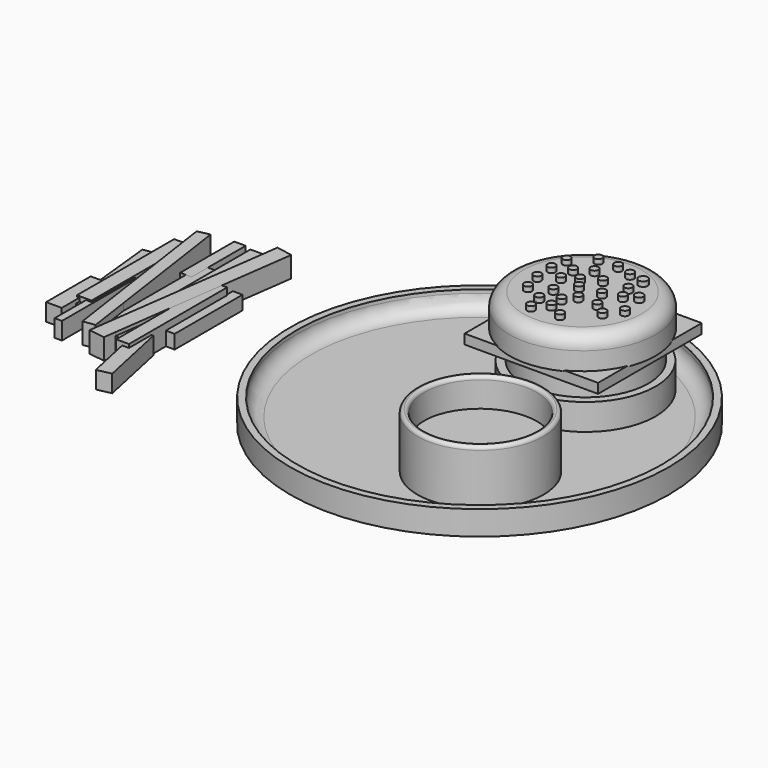
from build123d import *

# Parameters (mm, degrees)
F0_R      = 69.415848621
F1_DEPTH  = 8.89
F2_T      = -2.54
F3_R      = 5.08
F4_R      = 25.7769025516
F5_DEPTH  = 12.192
F6_R      = 22.9963503977
F7_DEPTH  = 19.05
F9_START  = 19.304
F8_W      = 48.926981166
F8_H      = 47.4879527465
F9_DEPTH  = 3.556
F11_START = 22.606
F10_R     = 26.7992090527
F11_DEPTH = 11.938
F12_R     = 5.08
F13_R     = 1.4675266157
F14_DEPTH = 36.322
F13_R_2   = 1.4390293509
F13_R_3   = 1.6781766258
F13_R_4   = 1.5498825968
F15_R     = 23.1464516615
F16_DEPTH = 22.606
F17_T     = 2.54
F18_R     = 21.0117914826
F19_DEPTH = 12.192
F20_R     = 1.26999
F22_DEPTH = 6.35
F21_W     = 0.3085602075
F21_H     = 28.0814692059
F23_DEPTH = 7.62
F24_DEPTH = 5.08
F25_DEPTH = 7.62
F26_DEPTH = 6.35
F21_W_2   = 2.106167376
F21_H_2   = 7.4712689966
F27_DEPTH = 5.08
F28_DEPTH = 5.08
F29_DEPTH = 7.62
F21_W_3   = 0.9008161724
F21_H_3   = 12.3305870922
F30_DEPTH = 6.858
F31_DEPTH = 6.35
F32_DEPTH = 5.08
F33_DEPTH = 6.35


# Not quite as in the source:
# - a fillet or chamfer is up to 0.001 mm smaller than in the source, because OpenCascade refuses the exact size
# - a shell that OpenCascade refuses in one call is made with other operations: the cavity is built on its own and cut out


with BuildPart() as f1:
    # F0 (on Top) → F1 (new body)
    with BuildSketch(Plane.XY):
        Circle(F0_R)
    extrude(amount=F1_DEPTH)

    # F2
    f2_openings = [f1.faces().sort_by_distance(p)[0] for p in [
        (0, 0, 8.89),
    ]]
    offset(amount=F2_T, openings=f2_openings)

    # F3
    f3_edges = [f1.edges().sort_by_distance(p)[0] for p in [
        (-66.875849, 0, 2.54),
    ]]
    fillet(f3_edges, radius=F3_R)

    # F4 (on Top) → F5 (join)
    with BuildSketch(Plane.XY):
        with Locations((13.4006887674, 31.7715257406)):
            Circle(F4_R)
    extrude(amount=F5_DEPTH)

    # F6 (on Top) → F7 (join)
    with BuildSketch(Plane.XY):
        with Locations((13.4006887674, 31.9251716137)):
            Circle(F6_R)
    extrude(amount=F7_DEPTH)

    # F15 (on Top) → F16 (join)
    with BuildSketch(Plane.XY):
        with Locations((21.2976261973, -26.1903237551)):
            Circle(F15_R)
    extrude(amount=F16_DEPTH)

    # F17: shell of thickness 2.54, made by hand


with BuildPart() as f9:
    # F8 (on Top) → F9 (new body)
    with BuildSketch(Plane.XY.offset(F9_START)):
        with Locations((13.2390661165, 30.9391203336)):
            Rectangle(F8_W, F8_H)
    extrude(amount=F9_DEPTH)


with BuildPart() as f11:
    # F10 (on Top) → F11 (new body)
    with BuildSketch(Plane.XY.offset(F11_START)):
        with Locations((13.0065530539, 30.9398267418)):
            Circle(F10_R)
    extrude(amount=F11_DEPTH)

    # F12
    f12_edges = [f11.edges().sort_by_distance(p)[0] for p in [
        (-13.792656, 30.939827, 34.544),
    ]]
    fillet(f12_edges, radius=F12_R)


with BuildPart() as f14:
    # F13 (on Top) → F14 (new body)
    with BuildSketch(Plane.XY):
        with Locations((0, 22.1610423177)):
            Circle(F13_R)
    extrude(amount=F14_DEPTH)


with BuildPart() as f14b:
    # F13 (on Top) → F14, piece 2 (new body)
    with BuildSketch(Plane.XY):
        with Locations((12.3756462708, 22.1610423177)):
            Circle(F13_R_2)
    extrude(amount=F14_DEPTH)


with BuildPart() as f14c:
    # F13 (on Top) → F14, piece 3 (new body)
    with BuildSketch(Plane.XY):
        with Locations((6.7634354346, 25.4012537548)):
            Circle(F13_R_2)
    extrude(amount=F14_DEPTH)


with BuildPart() as f14d:
    # F13 (on Top) → F14, piece 4 (new body)
    with BuildSketch(Plane.XY):
        with Locations((6.7634354346, 18.9208308807)):
            Circle(F13_R_2)
    extrude(amount=F14_DEPTH)


with BuildPart() as f14e:
    # F13 (on Top) → F14, piece 5 (new body)
    with BuildSketch(Plane.XY):
        with Locations((11.4056941927, 31.3545369015)):
            Circle(F13_R_2)
    extrude(amount=F14_DEPTH)


with BuildPart() as f14f:
    # F13 (on Top) → F14, piece 6 (new body)
    with BuildSketch(Plane.XY):
        with Locations((3.9288703727, 32.3982093437)):
            Circle(F13_R_2)
    extrude(amount=F14_DEPTH)


with BuildPart() as f14g:
    # F13 (on Top) → F14, piece 7 (new body)
    with BuildSketch(Plane.XY):
        with Locations((19.0983680662, 32.2760957669)):
            Circle(F13_R_2)
    extrude(amount=F14_DEPTH)


with BuildPart() as f14h:
    # F13 (on Top) → F14, piece 8 (new body)
    with BuildSketch(Plane.XY):
        with Locations((14.453937741, 38.4773673317)):
            Circle(F13_R_2)
    extrude(amount=F14_DEPTH)


with BuildPart() as f14i:
    # F13 (on Top) → F14, piece 9 (new body)
    with BuildSketch(Plane.XY):
        with Locations((15.2537068352, 26.1903237551)):
            Circle(F13_R_2)
    extrude(amount=F14_DEPTH)


with BuildPart() as f14j:
    # F13 (on Top) → F14, piece 10 (new body)
    with BuildSketch(Plane.XY):
        with Locations((22.4464706145, 25.903635466)):
            Circle(F13_R_2)
    extrude(amount=F14_DEPTH)


with BuildPart() as f14k:
    # F13 (on Top) → F14, piece 11 (new body)
    with BuildSketch(Plane.XY):
        with Locations((-2.0858600398, 35.5903968791)):
            Circle(F13_R_2)
    extrude(amount=F14_DEPTH)


with BuildPart() as f14l:
    # F13 (on Top) → F14, piece 12 (new body)
    with BuildSketch(Plane.XY):
        with Locations((-1.8430103329, 28.7853937772)):
            Circle(F13_R_2)
    extrude(amount=F14_DEPTH)


with BuildPart() as f14m:
    # F13 (on Top) → F14, piece 13 (new body)
    with BuildSketch(Plane.XY):
        with Locations((8.7462493805, 41.772702743)):
            Circle(F13_R_2)
    extrude(amount=F14_DEPTH)


with BuildPart() as f14n:
    # F13 (on Top) → F14, piece 14 (new body)
    with BuildSketch(Plane.XY):
        with Locations((8.7462493805, 35.1820319203)):
            Circle(F13_R_2)
    extrude(amount=F14_DEPTH)


with BuildPart() as f14o:
    # F13 (on Top) → F14, piece 15 (new body)
    with BuildSketch(Plane.XY):
        with Locations((3.6562509812, 38.3103937772)):
            Circle(F13_R_2)
    extrude(amount=F14_DEPTH)


with BuildPart() as f14p:
    # F13 (on Top) → F14, piece 16 (new body)
    with BuildSketch(Plane.XY):
        with Locations((-1.5703909413, 41.9232093437)):
            Circle(F13_R_2)
    extrude(amount=F14_DEPTH)


with BuildPart() as f14q:
    # F13 (on Top) → F14, piece 17 (new body)
    with BuildSketch(Plane.XY):
        with Locations((18.0482084397, 14.3602699913)):
            Circle(F13_R_2)
    extrude(amount=F14_DEPTH)


with BuildPart() as f14r:
    # F13 (on Top) → F14, piece 18 (new body)
    with BuildSketch(Plane.XY):
        with Locations((26.8960847251, 22.6954062536)):
            Circle(F13_R_2)
    extrude(amount=F14_DEPTH)


with BuildPart() as f14s:
    # F13 (on Top) → F14, piece 19 (new body)
    with BuildSketch(Plane.XY):
        with Locations((8.2464414958, 13.2429551706)):
            Circle(F13_R_2)
    extrude(amount=F14_DEPTH)


with BuildPart() as f14t:
    # F13 (on Top) → F14, piece 20 (new body)
    with BuildSketch(Plane.XY):
        with Locations((12.4221230696, 17.3662139487)):
            Circle(F13_R_2)
    extrude(amount=F14_DEPTH)


with BuildPart() as f14u:
    # F13 (on Top) → F14, piece 21 (new body)
    with BuildSketch(Plane.XY):
        with Locations((12.3846795339, 48.0746486285)):
            Circle(F13_R_2)
    extrude(amount=F14_DEPTH)


with BuildPart() as f14v:
    # F13 (on Top) → F14, piece 22 (new body)
    with BuildSketch(Plane.XY):
        with Locations((5.1078192271, 48.0746486285)):
            Circle(F13_R_2)
    extrude(amount=F14_DEPTH)


with BuildPart() as f14w:
    # F13 (on Top) → F14, piece 23 (new body)
    with BuildSketch(Plane.XY):
        with Locations((23.118837317, 39.3239505656)):
            Circle(F13_R_2)
    extrude(amount=F14_DEPTH)


with BuildPart() as f14x:
    # F13 (on Top) → F14, piece 24 (new body)
    with BuildSketch(Plane.XY):
        with Locations((18.053224942, 46.4046821027)):
            Circle(F13_R_2)
    extrude(amount=F14_DEPTH)


with BuildPart() as f14y:
    # F13 (on Top) → F14, piece 25 (new body)
    with BuildSketch(Plane.XY):
        with Locations((31.0522450493, 27.8401927665)):
            Circle(F13_R_2)
    extrude(amount=F14_DEPTH)


with BuildPart() as f14z:
    # F13 (on Top) → F14, piece 26 (new body)
    with BuildSketch(Plane.XY):
        with Locations((25.0722500137, 34.324733396)):
            Circle(F13_R_2)
    extrude(amount=F14_DEPTH)


with BuildPart() as f14ba:
    # F13 (on Top) → F14, piece 27 (new body)
    with BuildSketch(Plane.XY):
        with Locations((23.6000716686, 45.4733073711)):
            Circle(F13_R_3)
    extrude(amount=F14_DEPTH)


with BuildPart() as f14bb:
    # F13 (on Top) → F14, piece 28 (new body)
    with BuildSketch(Plane.XY):
        with Locations((29.0683787316, 36.8391387165)):
            Circle(F13_R_4)
    extrude(amount=F14_DEPTH)


with BuildPart() as f17_core1:
    # F17_t2: copy of F1
    add(f1.part)

    # the walls: a layer under each face that stays
    f17_faces = [f17_core1.faces().sort_by_distance(p)[0] for p in [
        (-66.875848621, 0, 8.255),
        (-65.3879510694, 0, 4.0278975516),
        (-64.7881253796, -18.5108929656, 8.89),
        (0, 0, 2.54),
        (-69.415848621, 0, 4.445),
        (-1.8488254641, -26.1903237551, 12.573),
        (-12.3762137841, 31.7715257406, 7.366),
        (0, 0, 0),
        (-3.7839129336, 14.5869240396, 12.192),
        (-9.5956616303, 31.9251716137, 15.621),
        (13.4006887674, 31.9251716137, 19.05),
    ]]
    thicken(f17_faces, amount=-F17_T, mode=Mode.SUBTRACT)

    # F17_s3 → F17_t4 (revolve, cut)
    with BuildSketch(Plane.XZ.offset(26.1903237551)):
        Polygon((44.4694778588, 2.5654), (44.4440778588, 0), (41.9040778588, 0), (41.9040778588, 2.54), align=None)
    revolve(axis=Axis((21.2976261973, -26.1903237551, 2.54), (0, 0, -1)), mode=Mode.SUBTRACT)

    # F17_s5 → F17_t6 (revolve, cut)
    with BuildSketch(Plane.XZ.offset(-31.7715257406)):
        Polygon((39.202991319, 2.5654), (39.177591319, 0), (36.637591319, 0), (36.637591319, 2.54), align=None)
    revolve(axis=Axis((13.4006887674, 31.7715257406, 2.54), (0, 0, -1)), mode=Mode.SUBTRACT)

    # F17_s7 → F17_t8 (revolve, cut)
    with BuildSketch(Plane.XZ.offset(-31.9251716137)):
        Polygon((36.4224391651, 12.2174), (36.3970391651, 9.652), (33.8570391651, 9.652), (33.8570391651, 12.192), align=None)
    revolve(axis=Axis((13.4006887674, 31.9251716137, 12.192), (0, 0, -1)), mode=Mode.SUBTRACT)


with BuildPart() as f1_1:
    add(f1.part)

    # what is left inside the walls is the cavity
    f17_cavity = [f17_core1.part.solids().sort_by_distance(p)[0] for p in [
        (0.716575, -26.190324, 15.917333),
        (13.400689, 24.025892, 2.5654),
    ]]
    add(f17_cavity, mode=Mode.SUBTRACT)

    # F18 (on Top) → F19 (join)
    with BuildSketch(Plane.XY):
        with Locations((21.5854309499, -26.8632397056)):
            Circle(F18_R)
    extrude(amount=F19_DEPTH)

    # F20 (radius 1.27 in the source; OpenCascade refuses exactly that, so slightly less here)
    f20_edges = [f1_1.edges().sort_by_distance(p)[0] for p in [
        (-1.848825, -26.190324, 22.606),
        (0.691175, -26.190324, 22.606),
    ]]
    fillet(f20_edges, radius=F20_R)


with BuildPart() as f22:
    # F21 (on face) → F22 (new body)
    with BuildSketch(Plane.XY.offset(2.54)):
        Polygon((-20.1991468536, -35.0447334349), (-16.6567120951, -51.5761016997), (-11.5006137639, -50.4712238908), (-17.0257425872, -24.6872799325), (-17.7025832236, -24.83210229), (-17.7025832236, -35.0447334349), align=None)
        Polygon((-22.1821762938, -25.7905926555), (-20.1991468536, -35.0447334349), (-17.7025832236, -35.0447334349), (-17.7025832236, -24.83210229), align=None)
    extrude(amount=F22_DEPTH)


with BuildPart() as f23:
    # F21 (on face) → F23 (new body)
    with BuildSketch(Plane.XY.offset(2.54)):
        Polygon((-22.3833005875, -35.0447334349), (-20.1991468536, -35.0447334349), (-22.1821762938, -25.7905926555), (-17.7025832236, -24.83210229), (-17.7025832236, -18.1428026408), (-18.0111434311, -18.1428026408), (-18.0111434311, 9.9386665651), (-19.6521536897, 9.9386665651), (-22.3833005875, -10.0328919954), align=None)
        Polygon((-22.1821762938, -25.7905926555), (-20.1991468536, -35.0447334349), (-17.7025832236, -35.0447334349), (-17.7025832236, -24.83210229), align=None)
        with Locations((-17.8568633273, -4.1020680379)):
            Rectangle(F21_W, F21_H)
        Polygon((-22.3833005875, 9.9386665651), (-22.3833005875, -10.0328919954), (-19.6521536897, 9.9386665651), align=None)
    extrude(amount=F23_DEPTH)


with BuildPart() as f24:
    # F21 (on face) → F24 (new body)
    with BuildSketch(Plane.XY.offset(2.54)):
        Polygon((-17.7025832236, 9.9386665651), (-17.7025832236, -18.1428026408), (-14.4805434311, -18.1428026408), (-14.4805434311, 12.9374377429), (-18.0111434311, 12.9374377429), (-18.0111434311, 9.9386665651), align=None)
        with Locations((-17.8568633273, -4.1020680379)):
            Rectangle(F21_W, F21_H)
    extrude(amount=F24_DEPTH)


with BuildPart() as f25:
    # F21 (on face) → F25 (new body)
    with BuildSketch(Plane.XY.offset(2.54)):
        Polygon((-25.9610270703, -36.1950782984), (-25.3534348722, -31.7520499229), (-28.7051629275, -31.7520499229), (-28.7051629275, -11.8827479087), (-30.0457645208, -21.6859200657), (-30.0457645208, -29.8663880676), (-31.1644583743, -29.8663880676), (-31.9185070693, -35.3803820908), align=None)
        Polygon((-25.3534348722, -31.7520499229), (-23.2695629275, -16.5137005657), (-23.2695629275, 27.8651703728), (-28.7051629275, -11.8827479087), (-28.7051629275, -31.7520499229), align=None)
        Polygon((-23.2695629275, -16.5137005657), (-22.3833005875, -10.0328919954), (-22.3833005875, 9.9386665651), (-19.6521536897, 9.9386665651), (-15.9358758894, 37.1140117557), (-21.854393352, 38.2136221794), (-23.2695629275, 27.8651703728), align=None)
        Polygon((-22.3833005875, 9.9386665651), (-22.3833005875, -10.0328919954), (-19.6521536897, 9.9386665651), align=None)
        Polygon((-30.0457645208, -29.8663880676), (-30.0457645208, -21.6859200657), (-31.1644583743, -29.8663880676), align=None)
    extrude(amount=F25_DEPTH)


with BuildPart() as f26:
    # F21 (on face) → F26 (new body)
    with BuildSketch(Plane.XY.offset(2.54)):
        Polygon((-23.2695629275, -31.7520499229), (-23.2695629275, -16.5137005657), (-25.3534348722, -31.7520499229), align=None)
        Polygon((-28.7051629275, -11.8827479087), (-23.2695629275, 27.8651703728), (-23.2695629275, 34.3817286193), (-28.7051629275, 34.3817286193), align=None)
        Polygon((-25.3534348722, -31.7520499229), (-23.2695629275, -16.5137005657), (-23.2695629275, 27.8651703728), (-28.7051629275, -11.8827479087), (-28.7051629275, -31.7520499229), align=None)
    extrude(amount=F26_DEPTH)


with BuildPart() as f27:
    # F21 (on face) → F27 (new body)
    with BuildSketch(Plane.XY.offset(2.54)):
        Polygon((-30.0457645208, -29.8663880676), (-30.0457645208, -21.6859200657), (-31.1644583743, -29.8663880676), align=None)
        Polygon((-34.8282344639, -29.8663880676), (-32.8429926838, -29.8663880676), (-34.8282344639, -16.1707288156), align=None)
        Polygon((-31.1644583743, -29.8663880676), (-30.0457645208, -21.6859200657), (-30.0457645208, 19.8916625232), (-32.7220670879, 19.8916625232), (-32.7220670879, 12.4203935266), (-34.8282344639, 12.4203935266), (-34.8282344639, -16.1707288156), (-32.8429926838, -29.8663880676), align=None)
        with Locations((-33.7751507759, 16.1560280249)):
            Rectangle(F21_W_2, F21_H_2)
    extrude(amount=F27_DEPTH)


with BuildPart() as f28:
    # F21 (on face) → F28 (new body)
    with BuildSketch(Plane.XY.offset(2.54)):
        with Locations((-33.7751507759, 16.1560280249)):
            Rectangle(F21_W_2, F21_H_2)
        Polygon((-34.8282344639, 19.8916625232), (-32.7220670879, 19.8916625232), (-32.7220670879, 37.2036620975), (-36.9220227003, 37.2036620975), (-36.9220227003, 12.4203935266), (-34.8282344639, 12.4203935266), align=None)
    extrude(amount=F28_DEPTH)


with BuildPart() as f29:
    # F21 (on face) → F29 (new body)
    with BuildSketch(Plane.XY.offset(2.54)):
        Polygon((-32.5698964298, -31.7504070699), (-32.8429926838, -29.8663880676), (-34.8282344639, -29.8663880676), (-34.8282344639, -16.1707288156), (-41.8996177614, 32.6128788292), (-46.2558828294, 31.6448174417), (-45.284405441, 24.9809194356), (-43.8396967947, 24.9809194356), (-43.8396967947, 15.0708678151), (-36.9220227003, -32.3812655591), align=None)
        Polygon((-45.284405441, 24.9809194356), (-43.8396967947, 15.0708678151), (-43.8396967947, 24.9809194356), align=None)
        Polygon((-34.8282344639, -29.8663880676), (-32.8429926838, -29.8663880676), (-34.8282344639, -16.1707288156), align=None)
    extrude(amount=F29_DEPTH)


with BuildPart() as f30:
    # F21 (on face) → F30 (new body)
    with BuildSketch(Plane.XY.offset(2.54)):
        Polygon((-45.284405441, 24.9809194356), (-43.8396967947, 15.0708678151), (-43.8396967947, 24.9809194356), align=None)
        Polygon((-43.8396967947, -0.0977143622), (-43.8396967947, 15.0708678151), (-45.284405441, 24.9809194356), (-49.1640232503, 24.9809194356), (-49.1640232503, 10.3856186005), (-45.8570056925, -17.4654246701), (-45.8477670327, -0.3904551618), align=None)
        Polygon((-45.8570056925, -17.4654246701), (-49.1640232503, 10.3856186005), (-49.1640232503, -7.2192241668), (-48.263207078, -7.2192241668), (-48.263207078, -19.5498112589), (-45.85813348, -19.5498112589), align=None)
        with Locations((-48.7136151642, -13.3845177128)):
            Rectangle(F21_W_3, F21_H_3)
        Polygon((-43.8396967947, -19.5498112589), (-43.8396967947, -0.0977143622), (-45.8477670327, -0.3904551618), (-45.8570056925, -17.4654246701), (-45.6095067755, -19.5498112589), align=None)
        Polygon((-45.85813348, -19.5498112589), (-45.6095067755, -19.5498112589), (-45.8570056925, -17.4654246701), align=None)
    extrude(amount=F30_DEPTH)


with BuildPart() as f31:
    # F21 (on face) → F31 (new body)
    with BuildSketch(Plane.XY.offset(2.54)):
        Polygon((-43.1694202125, 0), (-43.8396967947, -0.0977143622), (-43.8396967947, -19.5498112589), (-45.6095067755, -19.5498112589), (-45.4606637627, -20.80333747), (-45.8588372995, -20.8506163767), (-45.865919441, -33.9398905635), (-43.1694202125, -33.9398905635), align=None)
        Polygon((-43.8396967947, -19.5498112589), (-43.8396967947, -0.0977143622), (-45.8477670327, -0.3904551618), (-45.8570056925, -17.4654246701), (-45.6095067755, -19.5498112589), align=None)
        Polygon((-45.4606637627, -20.80333747), (-45.6095067755, -19.5498112589), (-45.85813348, -19.5498112589), (-45.8588372995, -20.8506163767), align=None)
        Polygon((-45.85813348, -19.5498112589), (-45.6095067755, -19.5498112589), (-45.8570056925, -17.4654246701), align=None)
    extrude(amount=F31_DEPTH)


with BuildPart() as f32:
    # F21 (on face) → F32 (new body)
    with BuildSketch(Plane.XY.offset(2.54)):
        Polygon((-49.1640232503, -7.2192241668), (-49.1640232503, 10.3856186005), (-50.0211715698, 17.6043510437), (-54.3451681733, 16.8895851821), (-51.8086992332, -7.2192241668), align=None)
        Polygon((-45.8570056925, -17.4654246701), (-49.1640232503, 10.3856186005), (-49.1640232503, -7.2192241668), (-48.263207078, -7.2192241668), (-48.263207078, -19.5498112589), (-45.85813348, -19.5498112589), align=None)
        with Locations((-48.7136151642, -13.3845177128)):
            Rectangle(F21_W_3, F21_H_3)
        Polygon((-49.1640232503, -19.5498112589), (-49.1640232503, -7.2192241668), (-51.8086992332, -7.2192241668), (-50.318834692, -21.3801940138), (-48.263207078, -21.1361099216), (-48.263207078, -19.5498112589), align=None)
        Polygon((-45.8588372995, -20.8506163767), (-45.85813348, -19.5498112589), (-48.263207078, -19.5498112589), (-48.263207078, -21.1361099216), align=None)
        Polygon((-45.4606637627, -20.80333747), (-45.6095067755, -19.5498112589), (-45.85813348, -19.5498112589), (-45.8588372995, -20.8506163767), align=None)
        Polygon((-45.85813348, -19.5498112589), (-45.6095067755, -19.5498112589), (-45.8570056925, -17.4654246701), align=None)
    extrude(amount=F32_DEPTH)


with BuildPart() as f33:
    # F21 (on face) → F33 (new body)
    with BuildSketch(Plane.XY.offset(2.54)):
        Polygon((-50.318834692, -21.3801940138), (-51.8086992332, -7.2192241668), (-54.0043227375, -7.2192241668), (-54.0043227375, -27.6662241668), (-48.263207078, -27.6662241668), (-48.263207078, -21.1361099216), align=None)
        Polygon((-49.1640232503, -19.5498112589), (-49.1640232503, -7.2192241668), (-51.8086992332, -7.2192241668), (-50.318834692, -21.3801940138), (-48.263207078, -21.1361099216), (-48.263207078, -19.5498112589), align=None)
        with Locations((-48.7136151642, -13.3845177128)):
            Rectangle(F21_W_3, F21_H_3)
    extrude(amount=F33_DEPTH)


with BuildPart() as f24_1:
    # F34: moved
    add(f24.part.moved(Location((-82.804, 0, -2.54))))


with BuildPart() as f23_1:
    # F34: moved
    add(f23.part.moved(Location((-82.804, 0, -2.54))))


with BuildPart() as f22_1:
    # F34: moved
    add(f22.part.moved(Location((-82.804, 0, -2.54))))


with BuildPart() as f25_1:
    # F34: moved
    add(f25.part.moved(Location((-82.804, 0, -2.54))))


with BuildPart() as f26_1:
    # F34: moved
    add(f26.part.moved(Location((-82.804, 0, -2.54))))


with BuildPart() as f27_1:
    # F34: moved
    add(f27.part.moved(Location((-82.804, 0, -2.54))))


with BuildPart() as f28_1:
    # F34: moved
    add(f28.part.moved(Location((-82.804, 0, -2.54))))


with BuildPart() as f29_1:
    # F34: moved
    add(f29.part.moved(Location((-82.804, 0, -2.54))))


with BuildPart() as f30_1:
    # F34: moved
    add(f30.part.moved(Location((-82.804, 0, -2.54))))


with BuildPart() as f32_1:
    # F34: moved
    add(f32.part.moved(Location((-82.804, 0, -2.54))))


with BuildPart() as f33_1:
    # F34: moved
    add(f33.part.moved(Location((-82.804, 0, -2.54))))


with BuildPart() as f31_1:
    # F34: moved
    add(f31.part.moved(Location((-82.804, 0, -2.54))))


solid = Compound([f9.part, f11.part, f14.part, f14b.part, f14c.part, f14d.part, f14e.part, f14f.part, f14g.part, f14h.part, f14i.part, f14j.part, f14k.part, f14l.part, f14m.part, f14n.part, f14o.part, f14p.part, f14q.part, f14r.part, f14s.part, f14t.part, f14u.part, f14v.part, f14w.part, f14x.part, f14y.part, f14z.part, f14ba.part, f14bb.part, f1_1.part, f24_1.part, f23_1.part, f22_1.part, f25_1.part, f26_1.part, f27_1.part, f28_1.part, f29_1.part, f30_1.part, f32_1.part, f33_1.part, f31_1.part])
